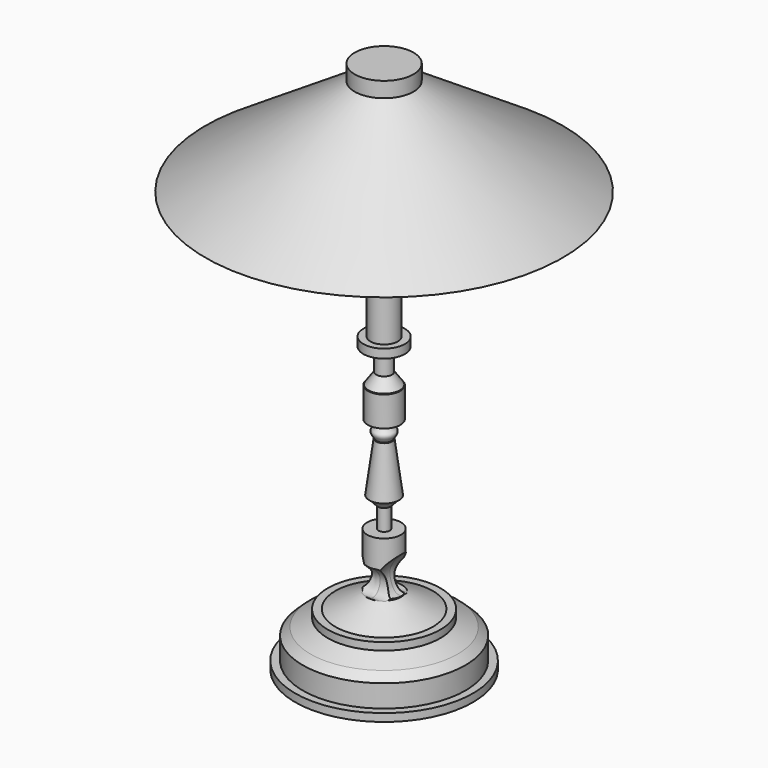
from build123d import *

# Parameters (mm, degrees)
F2_R      = 6.35
F3_DEPTH  = 46.5812087059
F5_DEPTH  = 12.7
F7_DEPTH  = 12.7
F8_R      = 2.1241867772
F9_DEPTH  = 8.0750538036
F15_DEPTH = 12.7
F16_DEPTH = 25.4
F19_DEPTH = 6.5224003047
F20_W     = 2.9630498029
F20_H     = 4.251010716
F22_R     = 5.1761447635
F23_DEPTH = 21.3190130889


# Not quite as in the source:
# - the program builds the solid bodies; features that only make, move or delete a surface that nothing else refers to are left out


with BuildPart() as f1:
    # F0 (on Right) → F1 (revolve)
    with BuildSketch(Plane.YZ):
        Polygon((-33.3996526897, 0), (0, 0), (0, 2.9368251562), (-30.5444467813, 2.9368251562), (-33.3996526897, 2.9368251562), align=None)
        Polygon((-30.5444467813, 2.9368251562), (0, 2.9368251562), (0, 29.2036384344), (-18.2930435985, 20.0245063752), (-21.1496353149, 20.0245063752), (-21.1496353149, 17.2138884664), (-27.6341680437, 14.0392314643), (-30.5444467813, 11.30739972), align=None)
    revolve(axis=Axis((0, 0, 14.6018192172), (0, 0, -1)))

    # F2 (on Top) → F3 (join)
    with BuildSketch(Plane.XY):
        Circle(F2_R)
    extrude(amount=F3_DEPTH)

    # F4 (on Front) → F5 (cut, symmetric)
    with BuildSketch(Plane.XZ):
        with BuildLine():
            Line((-6.5456423908, 39.9574637413), (-6.5013137646, 25.9207505733))
            add(Edge.make_bspline(
                [(-6.5013137646, 25.9207505733), (-5.9342158047, 26.4398288886), (-4.3830803487, 27.5506814233), (-3.2777647573, 30.2891836527), (-1.395448269, 35.8363896927), (-5.0464448383, 38.4652762696), (-6.5456423908, 39.9574637413)],
                knots=[0, 0, 0, 0, 0.1969965719, 0.4131278536, 0.6930587929, 1, 1, 1, 1], degree=3))
        make_face()
        with BuildLine():
            add(Edge.make_bspline(
                [(6.91843134, 25.9356857837), (6.4615811362, 26.4317820316), (4.3765860445, 26.16212875), (2.4003572787, 29.7084204211), (1.6204562499, 35.2264562182), (5.4215243853, 39.0932570962), (6.7391599528, 40.4120127497)],
                knots=[0, 0, 0, 0, 0.1797748395, 0.4078048421, 0.6857099785, 1, 1, 1, 1], degree=3))
            Line((6.91843134, 25.9356857837), (6.7391599528, 40.4120127497))
        make_face()
    extrude(amount=F5_DEPTH, both=True, mode=Mode.SUBTRACT)

    # F6 (on Right) → F7 (cut, symmetric)
    with BuildSketch(Plane.YZ):
        with BuildLine():
            add(Edge.make_bspline(
                [(-5.8341464028, 25.9447693825), (-5.3924653145, 25.9595849639), (-4.2969981453, 25.6598732134), (-1.9013328866, 27.8309508056), (-1.5663028536, 32.191785008), (-4.391798527, 34.5715170438), (-7.4715147679, 38.2651776178), (-7.7558497577, 25.441546686), (-6.2302875259, 25.9314813762), (-5.8341464028, 25.9447693825)],
                knots=[0, 0, 0, 0, 0.0947930762, 0.2298770407, 0.3882974273, 0.5472827147, 0.6657642898, 0.9149806576, 1, 1, 1, 1], degree=3))
        make_face()
        with BuildLine():
            add(Edge.make_bspline(
                [(3.5974502098, 25.8459635079), (2.9621780956, 25.8670793721), (2.0341545527, 25.7292806874), (1.7501776355, 28.395042234), (1.6315277997, 32.2131620822), (4.0347146423, 34.7973327197), (7.6276264347, 37.4629339024), (9.1122010123, 25.1206726587), (4.6862712184, 25.8097720931), (3.5974502098, 25.8459635079)],
                knots=[0, 0, 0, 0, 0.0883177345, 0.2023920431, 0.3526612548, 0.4992225418, 0.6205014506, 0.8486283239, 1, 1, 1, 1], degree=3))
        make_face()
    extrude(amount=F7_DEPTH, both=True, mode=Mode.SUBTRACT)

    # F8 (on face) → F9 (join)
    with BuildSketch(Plane.XY.offset(46.5812087059)):
        Circle(F8_R)
    extrude(amount=F9_DEPTH)

    # F10 (on Right) → F11 (revolve)
    with BuildSketch(Plane.YZ):
        Polygon((0, 57.5296916068), (0, 54.5936301351), (2.3989751935, 54.5936301351), (5.1056295633, 57.5296916068), align=None)
    revolve(axis=Axis((0, 0, 56.0616608709), (0, 0, -1)))


with BuildPart() as f13:
    # F12 (on Right) → F13 (revolve)
    with BuildSketch(Plane.YZ):
        Polygon((0, 99.5930209756), (0, 57.7275454998), (5.5517730211, 57.7275454998), align=None)
    revolve(axis=Axis((0, 0, 78.6602832377), (0, 0, 1)))

    # F14 (on Right) → F15 (cut, symmetric)
    with BuildSketch(Plane.YZ):
        Polygon((-3.3006183803, 76.3864517212), (3.273058217, 76.3864517212), (3.273058217, 77.0646333694), (-3.0602797323, 77.0646333694), align=None)
    extrude(amount=F15_DEPTH, both=True, mode=Mode.SUBTRACT)

    # F16 (cut): a face of the model
    f16_faces = [f13.faces().sort_by_distance(p)[0] for p in [
        (0, 0, 77.0646333694),
    ]]
    extrude(f16_faces, amount=-F16_DEPTH, mode=Mode.SUBTRACT)


with BuildPart() as f18:
    # F17 (on Right) → F18 (revolve)
    with BuildSketch(Plane.YZ):
        with BuildLine():
            Line((0, 76.2046277523), (2.6409111451, 76.2721374631))
            add(Edge.make_bspline(
                [(2.6409111451, 76.2721374631), (3.4488864302, 77.3281002381), (4.9381283593, 79.2744277102), (1.1591865232, 81.3879370989), (4.3117293958, 82.3002493652), (6.096187979, 82.8166529536)],
                knots=[0, 0, 0, 0, 0.3397919916, 0.6262970419, 1, 1, 1, 1], degree=3))
            Line((6.096187979, 82.8166529536), (6.096187979, 100.5699932575))
            Line((6.096187979, 100.5699932575), (0, 100.5699932575))
            Line((0, 100.5699932575), (0, 76.2046277523))
        make_face()
    revolve(axis=Axis((0, 0, 88.3873105049), (0, 0, -1)))

    # F19 (cut): a face of the model
    f19_faces = [f18.faces().sort_by_distance(p)[0] for p in [
        (0, 0, 100.5699932575),
    ]]
    extrude(f19_faces, amount=-F19_DEPTH, mode=Mode.SUBTRACT)

    # F20 (on Right) → F21 (revolve)
    with BuildSketch(Plane.YZ):
        Polygon((0, 93.5608744621), (5.9260996059, 94.2420065403), (2.9630498029, 98.4065532684), (0, 102.5710999966), align=None)
        Polygon((0, 102.5710999966), (2.9630498029, 98.4065532684), (2.9630498029, 102.5710999966), align=None)
        with Locations((1.4815249015, 104.6966053545)):
            Rectangle(F20_W, F20_H)
        Polygon((0, 110.1328134537), (0, 106.8221107125), (2.9630498029, 106.8221107125), (7.7988430858, 106.8221107125), (7.7988430858, 110.1328134537), align=None)
    revolve(axis=Axis((0, 0, 104.6966053545), (0, 0, 1)))

    # F22 (on face) → F23 (join)
    with BuildSketch(Plane.XY.offset(110.1328134537)):
        Circle(F22_R)
    extrude(amount=F23_DEPTH)


with BuildPart() as f25:
    # F24 (on Right) → F25 (revolve)
    with BuildSketch(Plane.YZ):
        with BuildLine():
            Line((0, 144.015327096), (0, 156.8502911308))
            add(Edge.make_bspline(
                [(0, 156.8502911308), (-8.6110368576, 156.8502911308), (-8.6110368576, 144.015327096), (-8.6110368576, 131.1803630612), (0, 131.1803630612)],
                knots=[0, 0, 0, 1.5707963268, 1.5707963268, 3.1415926536, 3.1415926536, 3.1415926536], degree=2, weights=[1, 0.7071067812, 1, 0.7071067812, 1]))
            Line((0, 131.1803630612), (0, 144.015327096))
        make_face()
    revolve(axis=Axis((0, 0, 144.015327096), (0, 0, 1)))


with BuildPart() as f27:
    # F26 (on Right) → F27 (revolve)
    with BuildSketch(Plane.YZ):
        Polygon((0, 200.3726363182), (0, 157.959997654), (16.4343323559, 157.959997654), (67.134976387, 157.959997654), (11.0505148768, 194.6172714233), (11.0505148768, 200.3726363182), align=None)
    revolve(axis=Axis((0, 0, 179.1663169861), (0, 0, -1)))


solid = Compound([f1.part, f13.part, f18.part, f25.part, f27.part])
